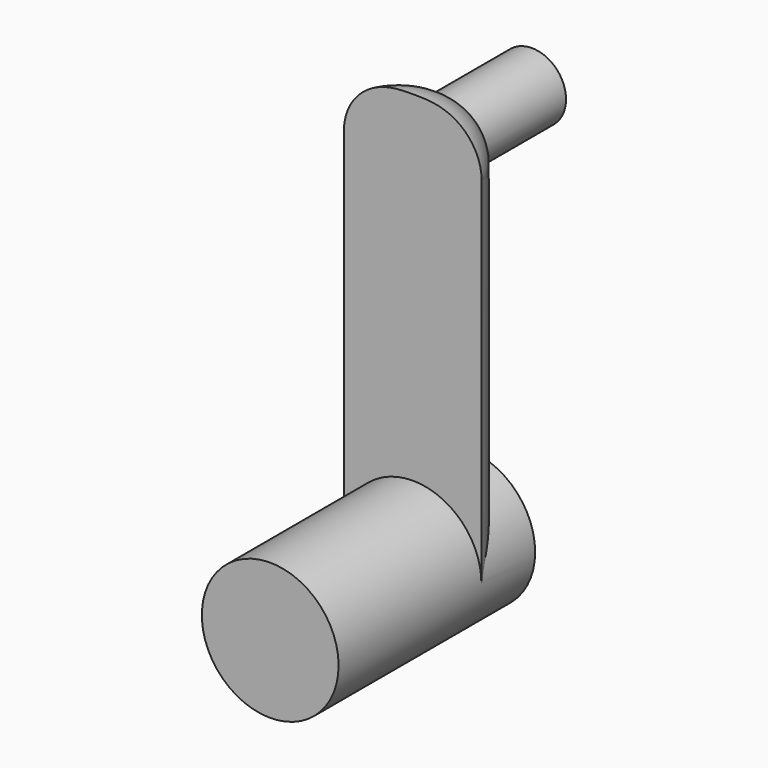
from build123d import *

# Parameters (mm, degrees)
F0_R        = 12.55
F1_DEPTH    = 45.1
F2_R        = 7.5
F3_DEPTH    = 3
F6_DEPTH    = 75
F7_T2_ANGLE = 359.64
F9_R        = 6.25
F10_DEPTH   = 25


# Not quite as in the source:
# - a fillet or chamfer that OpenCascade refuses, or shapes differently, is made with other operations: its cross-section is extruded or revolved along the edge and cut away or added


with BuildPart() as f1:
    # F0 (on Front) → F1 (new body)
    with BuildSketch(Plane.XZ):
        Circle(F0_R)
    extrude(amount=F1_DEPTH)

    # F2 (on Front) → F3 (join)
    with BuildSketch(Plane.XZ):
        Circle(F2_R)
    extrude(amount=-F3_DEPTH)

    # F4: fillet of radius 10 on 1 edges, made by hand

    # F4_s1 → F4_t2 (revolve, cut)
    with BuildSketch(Plane.XY):
        with BuildLine():
            ThreePointArc((7.5, 0), (4.2315549177, 2.2195444573), (0.3585715715, 3))
            Line((0.3585715715, 3), (7.5, 3))
            Line((7.5, 3), (7.5, 0))
        make_face()
    revolve(axis=Axis((0, 3, 0), (0, -1, 0)), mode=Mode.SUBTRACT)

    # F5 (on Top) → F6 (join)
    with BuildSketch(Plane.XY):
        with BuildLine():
            Line((-12.4928209826, -12.5774559094), (12.6060726016, -12.3417848491))
            ThreePointArc((12.6060726016, -12.3417848491), (-0.0335977446, -2.8508403226), (-12.4928209826, -12.5774559094))
        make_face()
    extrude(amount=F6_DEPTH)

    # F7: fillet of radius 10 on 1 edges, made by hand

    # F7_s1 → F7_t2 (revolve, cut)
    with BuildSketch(Plane(origin=(-0.1101500857, -0.0013803647, 0), x_dir=(0, 0, 1), z_dir=(-0.9999214878, -0.0125306879, 0))):
        with BuildLine():
            ThreePointArc((65, -28.8501313418), (72.0710678119, -25.9211991536), (75, -18.8501313418))
            Line((75, -18.8501313418), (75, -28.8501313418))
            Line((75, -28.8501313418), (65, -28.8501313418))
        make_face()
    revolve(axis=Axis((0.0884629639, -15.8502672786, 75), (0, 0, 1)), revolution_arc=F7_T2_ANGLE, mode=Mode.SUBTRACT)

    # F9 (on offset) → F10 (join)
    with BuildSketch(Plane.XZ.offset(10)):
        with Locations((-0.0335977446, 65)):
            Circle(F9_R)
    extrude(amount=-F10_DEPTH)


solid = f1.part
